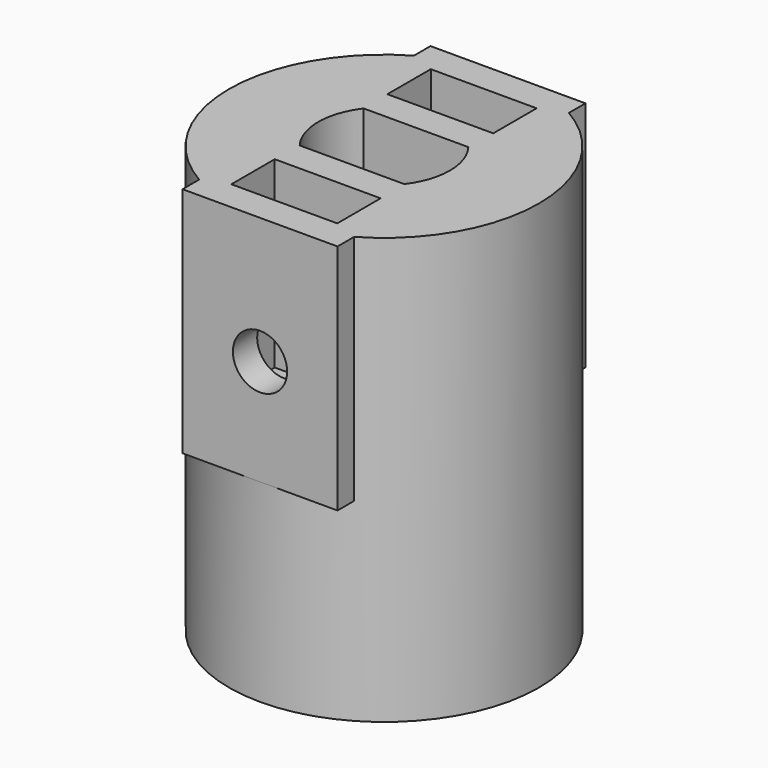
from build123d import *

# Parameters (mm, degrees)
F1_DEPTH = 90
F2_DEPTH = 75
F4_DEPTH = 90
F6_W     = 41
F6_H     = 21
F7_DEPTH = 71
F8_R     = 10.5
F9_DEPTH = 200


# Not quite as in the source:
# - a feature names something its author has since deleted; it is built from what else it names


with BuildPart() as f1:
    # F0 (on Top) → F1 (new body)
    with BuildSketch(Plane.XY):
        with BuildLine():
            ThreePointArc((30, -51.9615242271), (51.9615242271, -30), (60, 0))
            ThreePointArc((60, 0), (51.9615242271, 30), (30, 51.9615242271))
            ThreePointArc((30, 51.9615242271), (15.5291427062, 57.9555495773), (0, 60))
            ThreePointArc((0, 60), (-15.5291427062, 57.9555495773), (-30, 51.9615242271))
            ThreePointArc((-30, 51.9615242271), (-60, 0), (-30, -51.9615242271))
            ThreePointArc((-30, -51.9615242271), (-15.5291427062, -57.9555495773), (0, -60))
            ThreePointArc((0, -60), (15.5291427062, -57.9555495773), (30, -51.9615242271))
        make_face()
        with BuildLine():
            ThreePointArc((-8, 22.627416998), (0, 24), (8, 22.627416998))
            Line((8, 22.627416998), (8, 13))
            ThreePointArc((8, 13), (9.4644660941, 9.4644660941), (13, 8))
            Line((13, 8), (22.627416998, 8))
            ThreePointArc((22.627416998, 8), (24, 0), (22.627416998, -8))
            Line((22.627416998, -8), (13, -8))
            ThreePointArc((13, -8), (9.4644660941, -9.4644660941), (8, -13))
            Line((8, -13), (8, -22.627416998))
            ThreePointArc((8, -22.627416998), (0, -24), (-8, -22.627416998))
            Line((-8, -22.627416998), (-8, -13))
            ThreePointArc((-8, -13), (-9.4644660941, -9.4644660941), (-13, -8))
            Line((-13, -8), (-22.627416998, -8))
            ThreePointArc((-22.627416998, -8), (-24, 0), (-22.627416998, 8))
            Line((-22.627416998, 8), (-13, 8))
            ThreePointArc((-13, 8), (-9.4644660941, 9.4644660941), (-8, 13))
            Line((-8, 13), (-8, 22.627416998))
        make_face(mode=Mode.SUBTRACT)
        with BuildLine():
            ThreePointArc((0, 60), (15.5291427062, 57.9555495773), (30, 51.9615242271))
            Line((30, 51.9615242271), (30, 60))
            Line((30, 60), (0, 60))
        make_face()
        with BuildLine():
            Line((30, -60), (30, -51.9615242271))
            ThreePointArc((30, -51.9615242271), (15.5291427062, -57.9555495773), (0, -60))
            Line((0, -60), (30, -60))
        make_face()
        with BuildLine():
            ThreePointArc((-30, 51.9615242271), (-15.5291427062, 57.9555495773), (0, 60))
            Line((0, 60), (-30, 60))
            Line((-30, 60), (-30, 51.9615242271))
        make_face()
        with BuildLine():
            Line((-30, -60), (0, -60))
            ThreePointArc((0, -60), (-15.5291427062, -57.9555495773), (-30, -51.9615242271))
            Line((-30, -51.9615242271), (-30, -60))
        make_face()
        with BuildLine():
            Line((8, 13), (8, 22.627416998))
            ThreePointArc((8, 22.627416998), (0, 24), (-8, 22.627416998))
            Line((-8, 22.627416998), (-8, 13))
            ThreePointArc((-8, 13), (-9.4644660941, 9.4644660941), (-13, 8))
            Line((-13, 8), (-22.627416998, 8))
            ThreePointArc((-22.627416998, 8), (-24, 0), (-22.627416998, -8))
            Line((-22.627416998, -8), (-13, -8))
            ThreePointArc((-13, -8), (-9.4644660941, -9.4644660941), (-8, -13))
            Line((-8, -13), (-8, -22.627416998))
            ThreePointArc((-8, -22.627416998), (0, -24), (8, -22.627416998))
            Line((8, -22.627416998), (8, -13))
            ThreePointArc((8, -13), (9.4644660941, -9.4644660941), (13, -8))
            Line((13, -8), (22.627416998, -8))
            ThreePointArc((22.627416998, -8), (24, 0), (22.627416998, 8))
            Line((22.627416998, 8), (13, 8))
            ThreePointArc((13, 8), (9.4644660941, 9.4644660941), (8, 13))
        make_face()
    extrude(amount=F1_DEPTH)

    # F0 (on Top) → F2 (join)
    with BuildSketch(Plane.XY):
        with BuildLine():
            ThreePointArc((30, -51.9615242271), (51.9615242271, -30), (60, 0))
            ThreePointArc((60, 0), (51.9615242271, 30), (30, 51.9615242271))
            ThreePointArc((30, 51.9615242271), (15.5291427062, 57.9555495773), (0, 60))
            ThreePointArc((0, 60), (-15.5291427062, 57.9555495773), (-30, 51.9615242271))
            ThreePointArc((-30, 51.9615242271), (-60, 0), (-30, -51.9615242271))
            ThreePointArc((-30, -51.9615242271), (-15.5291427062, -57.9555495773), (0, -60))
            ThreePointArc((0, -60), (15.5291427062, -57.9555495773), (30, -51.9615242271))
        make_face()
        with BuildLine():
            ThreePointArc((-8, 22.627416998), (0, 24), (8, 22.627416998))
            Line((8, 22.627416998), (8, 13))
            ThreePointArc((8, 13), (9.4644660941, 9.4644660941), (13, 8))
            Line((13, 8), (22.627416998, 8))
            ThreePointArc((22.627416998, 8), (24, 0), (22.627416998, -8))
            Line((22.627416998, -8), (13, -8))
            ThreePointArc((13, -8), (9.4644660941, -9.4644660941), (8, -13))
            Line((8, -13), (8, -22.627416998))
            ThreePointArc((8, -22.627416998), (0, -24), (-8, -22.627416998))
            Line((-8, -22.627416998), (-8, -13))
            ThreePointArc((-8, -13), (-9.4644660941, -9.4644660941), (-13, -8))
            Line((-13, -8), (-22.627416998, -8))
            ThreePointArc((-22.627416998, -8), (-24, 0), (-22.627416998, 8))
            Line((-22.627416998, 8), (-13, 8))
            ThreePointArc((-13, 8), (-9.4644660941, 9.4644660941), (-8, 13))
            Line((-8, 13), (-8, 22.627416998))
        make_face(mode=Mode.SUBTRACT)
    extrude(amount=-F2_DEPTH)

    # F3 (on face) → F4 (cut)
    with BuildSketch(Plane.XY.offset(90)):
        with BuildLine():
            ThreePointArc((20.2484567313, -15.5), (24.1514559256, -8.1827365029), (25.5, 0))
            ThreePointArc((25.5, 0), (24.1514559256, 8.1827365029), (20.2484567313, 15.5))
            Line((20.2484567313, 15.5), (-20.2484567313, 15.5))
            ThreePointArc((-20.2484567313, 15.5), (-25.5, 0), (-20.2484567313, -15.5))
            Line((-20.2484567313, -15.5), (20.2484567313, -15.5))
        make_face()
    extrude(amount=-F4_DEPTH, mode=Mode.SUBTRACT)

    # F6 (on face) → F7 (cut)
    with BuildSketch(Plane.XY.offset(90)):
        with Locations((0, 37.75)):
            Rectangle(F6_W, F6_H)
        with Locations((0, -37.75)):
            Rectangle(F6_W, F6_H)
    extrude(amount=-F7_DEPTH, mode=Mode.SUBTRACT)

    # F8 (on face) → F9 (cut)
    with BuildSketch(Plane(origin=(0, 60, 0), x_dir=(-1, 0, 0), z_dir=(0, 1, 0))):
        with Locations((0, 41)):
            Circle(F8_R)
    extrude(amount=-F9_DEPTH, mode=Mode.SUBTRACT)


solid = f1.part
